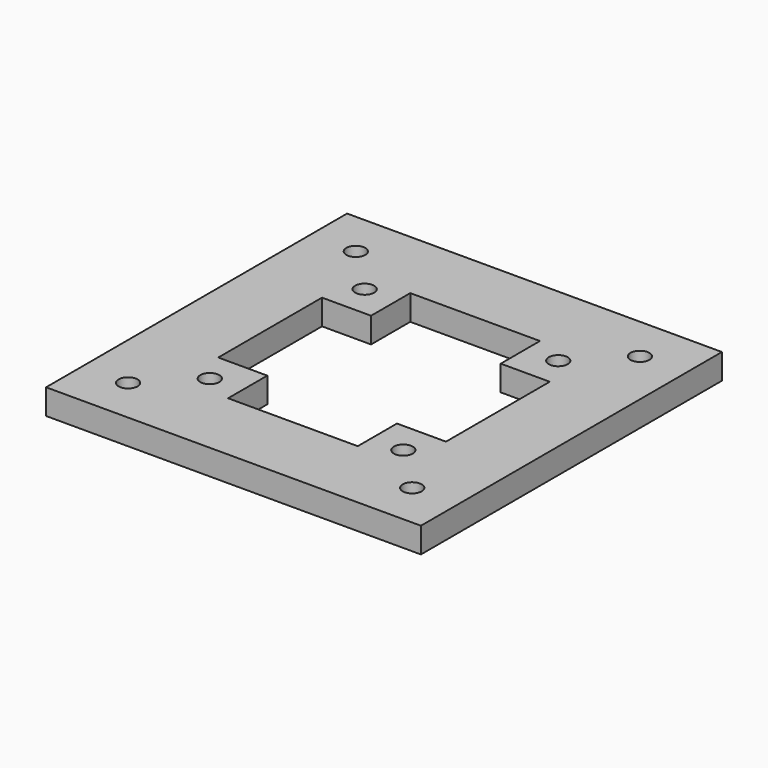
from build123d import *

# Parameters (mm, degrees)
F1_DEPTH = 2
F2_DEPTH = 4


with BuildPart() as f1:
    # F0 (on Top) → F1 (new body)
    with BuildSketch(Plane.XY):
        Polygon((0, -7.75), (0, -43.674267101), (7.675, -43.674267101), (7.675, -36), (7.675, -25.75), (7.675, -15.5), (7.675, -7.75), align=None)
        with BuildLine():
            Line((0, 0), (0, -7.75))
            Line((0, -7.75), (7.675, -7.75))
            Line((7.675, -7.75), (4.2740389016, -4.3158047541))
            ThreePointArc((4.2740389016, -4.3158047541), (2.152743633, -4.3054905145), (2.1630578726, -2.1841952459))
            Line((2.1630578726, -2.1841952459), (0, 0))
        make_face()
        with BuildLine():
            Line((7.675, 0), (0, 0))
            Line((0, 0), (2.1630578726, -2.1841952459))
            ThreePointArc((2.1630578726, -2.1841952459), (3.7959409001, -1.8655803072), (4.7185483871, -3.25))
            ThreePointArc((4.7185483871, -3.25), (4.6029680799, -3.827392513), (4.2740389016, -4.3158047541))
            Line((4.2740389016, -4.3158047541), (7.675, -7.75))
            Line((7.675, -7.75), (7.675, 0))
        make_face()
        Polygon((7.675, 0), (7.675, -7.75), (15.425, -7.75), (25.675, -7.75), (35.925, -7.75), (43.6, -7.75), (43.6, 0), align=None)
        Polygon((43.675, -36), (43.675, -43.75), (51.35, -43.75), (51.35, -7.825732899), (43.675, -7.825732899), (43.675, -15.5), (43.675, -25.75), align=None)
        Polygon((43.6, -7.825732899), (43.675, -7.825732899), (43.675, -7.75), (43.6, -7.825), align=None)
        with BuildLine():
            Line((51.35, -7.825732899), (51.35, 0))
            Line((51.35, 0), (49.1869421274, -2.1841952459))
            ThreePointArc((49.1869421274, -2.1841952459), (49.5158713057, -2.672607487), (49.6314516129, -3.25))
            ThreePointArc((49.6314516129, -3.25), (48.7088441259, -4.6344196928), (47.0759610984, -4.3158047541))
            Line((47.0759610984, -4.3158047541), (43.675, -7.75))
            Line((43.675, -7.75), (43.675, -7.825732899))
            Line((43.675, -7.825732899), (51.35, -7.825732899))
        make_face()
        with BuildLine():
            Line((49.1869421274, -2.1841952459), (51.35, 0))
            Line((51.35, 0), (43.6, 0))
            Line((43.6, 0), (43.6, -7.75))
            Line((43.6, -7.75), (43.675, -7.75))
            Line((43.675, -7.75), (47.0759610984, -4.3158047541))
            ThreePointArc((47.0759610984, -4.3158047541), (47.0656468588, -2.1945094855), (49.1869421274, -2.1841952459))
        make_face()
        with BuildLine():
            Line((9.3143398282, -9.3893398282), (7.675, -7.75))
            Line((7.675, -7.75), (7.675, -15.5))
            Line((7.675, -15.5), (11.55, -11.625))
            Line((11.55, -11.625), (11.4356601718, -11.5106601718))
            ThreePointArc((11.4356601718, -11.5106601718), (9.3143398282, -11.5106601718), (9.3143398282, -9.3893398282))
        make_face()
        Polygon((11.55, -11.625), (7.675, -15.5), (15.425, -15.5), align=None)
        Polygon((15.425, -15.5), (15.425, -7.75), (11.55, -11.625), align=None)
        with BuildLine():
            Line((15.425, -7.75), (7.675, -7.75))
            Line((7.675, -7.75), (9.3143398282, -9.3893398282))
            ThreePointArc((9.3143398282, -9.3893398282), (10.9490251485, -9.0641807012), (11.875, -10.45))
            ThreePointArc((11.875, -10.45), (11.7608192988, -11.0240251485), (11.4356601718, -11.5106601718))
            Line((11.4356601718, -11.5106601718), (11.55, -11.625))
            Line((11.55, -11.625), (15.425, -7.75))
        make_face()
        Polygon((39.8, -39.875), (43.675, -36), (35.925, -36), align=None)
        Polygon((35.925, -36), (35.925, -43.75), (39.8, -39.875), align=None)
        with BuildLine():
            Line((35.925, -43.75), (43.675, -43.75))
            Line((43.675, -43.75), (42.0356601718, -42.1106601718))
            ThreePointArc((42.0356601718, -42.1106601718), (39.9143398282, -42.1106601718), (39.9143398282, -39.9893398282))
            Line((39.9143398282, -39.9893398282), (39.8, -39.875))
            Line((39.8, -39.875), (35.925, -43.75))
        make_face()
        Polygon((7.75, -43.75), (7.75, -51.5), (43.675, -51.5), (43.675, -43.75), (35.925, -43.75), (25.675, -43.75), (15.425, -43.75), align=None)
        with BuildLine():
            Line((42.0356601718, -42.1106601718), (43.675, -43.75))
            Line((43.675, -43.75), (43.675, -36))
            Line((43.675, -36), (39.8, -39.875))
            Line((39.8, -39.875), (39.9143398282, -39.9893398282))
            ThreePointArc((39.9143398282, -39.9893398282), (41.5490251485, -39.6641807012), (42.475, -41.05))
            ThreePointArc((42.475, -41.05), (42.3608192988, -41.6240251485), (42.0356601718, -42.1106601718))
        make_face()
        Polygon((7.675, -43.75), (7.75, -43.75), (7.75, -43.675), align=None)
        with BuildLine():
            Line((7.75, -43.675), (7.75, -43.75))
            Line((7.75, -43.75), (15.425, -43.75))
            Line((15.425, -43.75), (11.55, -39.875))
            Line((11.55, -39.875), (11.4356601718, -39.9893398282))
            ThreePointArc((11.4356601718, -39.9893398282), (11.7608192988, -40.4759748515), (11.875, -41.05))
            ThreePointArc((11.875, -41.05), (10.9490251485, -42.4358192988), (9.3143398282, -42.1106601718))
            Line((9.3143398282, -42.1106601718), (7.75, -43.675))
        make_face()
        Polygon((7.75, -43.674267101), (7.675, -43.674267101), (7.675, -43.75), (7.75, -43.675), align=None)
        with BuildLine():
            Line((7.675, -36), (7.675, -43.674267101))
            Line((7.675, -43.674267101), (7.75, -43.674267101))
            Line((7.75, -43.674267101), (7.75, -43.675))
            Line((7.75, -43.675), (9.3143398282, -42.1106601718))
            ThreePointArc((9.3143398282, -42.1106601718), (9.3143398282, -39.9893398282), (11.4356601718, -39.9893398282))
            Line((11.4356601718, -39.9893398282), (11.55, -39.875))
            Line((11.55, -39.875), (7.675, -36))
        make_face()
        with BuildLine():
            Line((0, -43.674267101), (0, -51.5))
            Line((0, -51.5), (2.1630578726, -49.3158047541))
            ThreePointArc((2.1630578726, -49.3158047541), (2.152743633, -47.1945094855), (4.2740389016, -47.1841952459))
            Line((4.2740389016, -47.1841952459), (7.675, -43.75))
            Line((7.675, -43.75), (7.675, -43.674267101))
            Line((7.675, -43.674267101), (0, -43.674267101))
        make_face()
        with BuildLine():
            Line((2.1630578726, -49.3158047541), (0, -51.5))
            Line((0, -51.5), (7.75, -51.5))
            Line((7.75, -51.5), (7.75, -43.75))
            Line((7.75, -43.75), (7.675, -43.75))
            Line((7.675, -43.75), (4.2740389016, -47.1841952459))
            ThreePointArc((4.2740389016, -47.1841952459), (4.6029680799, -47.672607487), (4.7185483871, -48.25))
            ThreePointArc((4.7185483871, -48.25), (3.7959409001, -49.6344196928), (2.1630578726, -49.3158047541))
        make_face()
        with BuildLine():
            Line((43.675, -43.75), (43.675, -51.5))
            Line((43.675, -51.5), (51.35, -51.5))
            Line((51.35, -51.5), (49.1869421274, -49.3158047541))
            ThreePointArc((49.1869421274, -49.3158047541), (47.0656468588, -49.3054905145), (47.0759610984, -47.1841952459))
            Line((47.0759610984, -47.1841952459), (43.675, -43.75))
        make_face()
        with BuildLine():
            Line((49.1869421274, -49.3158047541), (51.35, -51.5))
            Line((51.35, -51.5), (51.35, -43.75))
            Line((51.35, -43.75), (43.675, -43.75))
            Line((43.675, -43.75), (47.0759610984, -47.1841952459))
            ThreePointArc((47.0759610984, -47.1841952459), (48.7088441259, -46.8655803072), (49.6314516129, -48.25))
            ThreePointArc((49.6314516129, -48.25), (49.5158713057, -48.827392513), (49.1869421274, -49.3158047541))
        make_face()
        Polygon((15.425, -36), (7.675, -36), (11.55, -39.875), align=None)
        Polygon((11.55, -39.875), (15.425, -43.75), (15.425, -36), align=None)
        Polygon((39.8, -11.625), (35.925, -7.75), (35.925, -15.5), align=None)
        Polygon((35.925, -15.5), (43.675, -15.5), (39.8, -11.625), align=None)
        with BuildLine():
            Line((43.6, -7.825), (43.6, -7.75))
            Line((43.6, -7.75), (35.925, -7.75))
            Line((35.925, -7.75), (39.8, -11.625))
            Line((39.8, -11.625), (39.9143398282, -11.5106601718))
            ThreePointArc((39.9143398282, -11.5106601718), (39.9143398282, -9.3893398282), (42.0356601718, -9.3893398282))
            Line((42.0356601718, -9.3893398282), (43.6, -7.825))
        make_face()
        with BuildLine():
            Line((43.675, -15.5), (43.675, -7.825732899))
            Line((43.675, -7.825732899), (43.6, -7.825732899))
            Line((43.6, -7.825732899), (43.6, -7.825))
            Line((43.6, -7.825), (42.0356601718, -9.3893398282))
            ThreePointArc((42.0356601718, -9.3893398282), (42.3608192988, -9.8759748515), (42.475, -10.45))
            ThreePointArc((42.475, -10.45), (41.5490251485, -11.8358192988), (39.9143398282, -11.5106601718))
            Line((39.9143398282, -11.5106601718), (39.8, -11.625))
            Line((39.8, -11.625), (43.675, -15.5))
        make_face()
    extrude(amount=F1_DEPTH)

    # F0 (on Top) → F2 (join)
    with BuildSketch(Plane.XY):
        with BuildLine():
            Line((2.1630578726, -49.3158047541), (0, -51.5))
            Line((0, -51.5), (7.75, -51.5))
            Line((7.75, -51.5), (7.75, -43.75))
            Line((7.75, -43.75), (7.675, -43.75))
            Line((7.675, -43.75), (4.2740389016, -47.1841952459))
            ThreePointArc((4.2740389016, -47.1841952459), (4.6029680799, -47.672607487), (4.7185483871, -48.25))
            ThreePointArc((4.7185483871, -48.25), (3.7959409001, -49.6344196928), (2.1630578726, -49.3158047541))
        make_face()
        Polygon((-3.95, -55.4885993485), (0, -51.5), (0, -43.674267101), (0, -7.75), (0, 0), (-3.95, 3.9885993485), align=None)
        with BuildLine():
            Line((0, -43.674267101), (0, -51.5))
            Line((0, -51.5), (2.1630578726, -49.3158047541))
            ThreePointArc((2.1630578726, -49.3158047541), (2.152743633, -47.1945094855), (4.2740389016, -47.1841952459))
            Line((4.2740389016, -47.1841952459), (7.675, -43.75))
            Line((7.675, -43.75), (7.675, -43.674267101))
            Line((7.675, -43.674267101), (0, -43.674267101))
        make_face()
        Polygon((7.75, -51.5), (0, -51.5), (-3.95, -55.4885993485), (55.3, -55.4885993485), (51.35, -51.5), (43.675, -51.5), align=None)
        Polygon((7.75, -43.75), (7.75, -51.5), (43.675, -51.5), (43.675, -43.75), (35.925, -43.75), (25.675, -43.75), (15.425, -43.75), align=None)
        Polygon((0, -7.75), (0, -43.674267101), (7.675, -43.674267101), (7.675, -36), (7.675, -25.75), (7.675, -15.5), (7.675, -7.75), align=None)
        with BuildLine():
            Line((43.675, -43.75), (43.675, -51.5))
            Line((43.675, -51.5), (51.35, -51.5))
            Line((51.35, -51.5), (49.1869421274, -49.3158047541))
            ThreePointArc((49.1869421274, -49.3158047541), (47.0656468588, -49.3054905145), (47.0759610984, -47.1841952459))
            Line((47.0759610984, -47.1841952459), (43.675, -43.75))
        make_face()
        with BuildLine():
            Line((7.75, -43.675), (7.75, -43.75))
            Line((7.75, -43.75), (15.425, -43.75))
            Line((15.425, -43.75), (11.55, -39.875))
            Line((11.55, -39.875), (11.4356601718, -39.9893398282))
            ThreePointArc((11.4356601718, -39.9893398282), (11.7608192988, -40.4759748515), (11.875, -41.05))
            ThreePointArc((11.875, -41.05), (10.9490251485, -42.4358192988), (9.3143398282, -42.1106601718))
            Line((9.3143398282, -42.1106601718), (7.75, -43.675))
        make_face()
        Polygon((7.675, -43.75), (7.75, -43.75), (7.75, -43.675), align=None)
        with BuildLine():
            Line((0, 0), (0, -7.75))
            Line((0, -7.75), (7.675, -7.75))
            Line((7.675, -7.75), (4.2740389016, -4.3158047541))
            ThreePointArc((4.2740389016, -4.3158047541), (2.152743633, -4.3054905145), (2.1630578726, -2.1841952459))
            Line((2.1630578726, -2.1841952459), (0, 0))
        make_face()
        Polygon((7.75, -43.674267101), (7.675, -43.674267101), (7.675, -43.75), (7.75, -43.675), align=None)
        with BuildLine():
            Line((7.675, -36), (7.675, -43.674267101))
            Line((7.675, -43.674267101), (7.75, -43.674267101))
            Line((7.75, -43.674267101), (7.75, -43.675))
            Line((7.75, -43.675), (9.3143398282, -42.1106601718))
            ThreePointArc((9.3143398282, -42.1106601718), (9.3143398282, -39.9893398282), (11.4356601718, -39.9893398282))
            Line((11.4356601718, -39.9893398282), (11.55, -39.875))
            Line((11.55, -39.875), (7.675, -36))
        make_face()
        Polygon((51.35, -51.5), (55.3, -55.4885993485), (55.3, 3.9885993485), (51.35, 0), (51.35, -7.825732899), (51.35, -43.75), align=None)
        Polygon((55.3, 3.9885993485), (-3.95, 3.9885993485), (0, 0), (7.675, 0), (43.6, 0), (51.35, 0), align=None)
        with BuildLine():
            Line((49.1869421274, -49.3158047541), (51.35, -51.5))
            Line((51.35, -51.5), (51.35, -43.75))
            Line((51.35, -43.75), (43.675, -43.75))
            Line((43.675, -43.75), (47.0759610984, -47.1841952459))
            ThreePointArc((47.0759610984, -47.1841952459), (48.7088441259, -46.8655803072), (49.6314516129, -48.25))
            ThreePointArc((49.6314516129, -48.25), (49.5158713057, -48.827392513), (49.1869421274, -49.3158047541))
        make_face()
        with BuildLine():
            Line((42.0356601718, -42.1106601718), (43.675, -43.75))
            Line((43.675, -43.75), (43.675, -36))
            Line((43.675, -36), (39.8, -39.875))
            Line((39.8, -39.875), (39.9143398282, -39.9893398282))
            ThreePointArc((39.9143398282, -39.9893398282), (41.5490251485, -39.6641807012), (42.475, -41.05))
            ThreePointArc((42.475, -41.05), (42.3608192988, -41.6240251485), (42.0356601718, -42.1106601718))
        make_face()
        with BuildLine():
            Line((35.925, -43.75), (43.675, -43.75))
            Line((43.675, -43.75), (42.0356601718, -42.1106601718))
            ThreePointArc((42.0356601718, -42.1106601718), (39.9143398282, -42.1106601718), (39.9143398282, -39.9893398282))
            Line((39.9143398282, -39.9893398282), (39.8, -39.875))
            Line((39.8, -39.875), (35.925, -43.75))
        make_face()
        Polygon((43.675, -36), (43.675, -43.75), (51.35, -43.75), (51.35, -7.825732899), (43.675, -7.825732899), (43.675, -15.5), (43.675, -25.75), align=None)
        Polygon((11.55, -39.875), (15.425, -43.75), (15.425, -36), align=None)
        with BuildLine():
            Line((7.675, 0), (0, 0))
            Line((0, 0), (2.1630578726, -2.1841952459))
            ThreePointArc((2.1630578726, -2.1841952459), (3.7959409001, -1.8655803072), (4.7185483871, -3.25))
            ThreePointArc((4.7185483871, -3.25), (4.6029680799, -3.827392513), (4.2740389016, -4.3158047541))
            Line((4.2740389016, -4.3158047541), (7.675, -7.75))
            Line((7.675, -7.75), (7.675, 0))
        make_face()
        Polygon((7.675, 0), (7.675, -7.75), (15.425, -7.75), (25.675, -7.75), (35.925, -7.75), (43.6, -7.75), (43.6, 0), align=None)
        with BuildLine():
            Line((9.3143398282, -9.3893398282), (7.675, -7.75))
            Line((7.675, -7.75), (7.675, -15.5))
            Line((7.675, -15.5), (11.55, -11.625))
            Line((11.55, -11.625), (11.4356601718, -11.5106601718))
            ThreePointArc((11.4356601718, -11.5106601718), (9.3143398282, -11.5106601718), (9.3143398282, -9.3893398282))
        make_face()
        with BuildLine():
            Line((15.425, -7.75), (7.675, -7.75))
            Line((7.675, -7.75), (9.3143398282, -9.3893398282))
            ThreePointArc((9.3143398282, -9.3893398282), (10.9490251485, -9.0641807012), (11.875, -10.45))
            ThreePointArc((11.875, -10.45), (11.7608192988, -11.0240251485), (11.4356601718, -11.5106601718))
            Line((11.4356601718, -11.5106601718), (11.55, -11.625))
            Line((11.55, -11.625), (15.425, -7.75))
        make_face()
        Polygon((15.425, -36), (7.675, -36), (11.55, -39.875), align=None)
        Polygon((35.925, -36), (35.925, -43.75), (39.8, -39.875), align=None)
        Polygon((39.8, -39.875), (43.675, -36), (35.925, -36), align=None)
        Polygon((15.425, -15.5), (15.425, -7.75), (11.55, -11.625), align=None)
        Polygon((11.55, -11.625), (7.675, -15.5), (15.425, -15.5), align=None)
        with BuildLine():
            Line((49.1869421274, -2.1841952459), (51.35, 0))
            Line((51.35, 0), (43.6, 0))
            Line((43.6, 0), (43.6, -7.75))
            Line((43.6, -7.75), (43.675, -7.75))
            Line((43.675, -7.75), (47.0759610984, -4.3158047541))
            ThreePointArc((47.0759610984, -4.3158047541), (47.0656468588, -2.1945094855), (49.1869421274, -2.1841952459))
        make_face()
        with BuildLine():
            Line((51.35, -7.825732899), (51.35, 0))
            Line((51.35, 0), (49.1869421274, -2.1841952459))
            ThreePointArc((49.1869421274, -2.1841952459), (49.5158713057, -2.672607487), (49.6314516129, -3.25))
            ThreePointArc((49.6314516129, -3.25), (48.7088441259, -4.6344196928), (47.0759610984, -4.3158047541))
            Line((47.0759610984, -4.3158047541), (43.675, -7.75))
            Line((43.675, -7.75), (43.675, -7.825732899))
            Line((43.675, -7.825732899), (51.35, -7.825732899))
        make_face()
        Polygon((43.6, -7.825732899), (43.675, -7.825732899), (43.675, -7.75), (43.6, -7.825), align=None)
        with BuildLine():
            Line((43.675, -15.5), (43.675, -7.825732899))
            Line((43.675, -7.825732899), (43.6, -7.825732899))
            Line((43.6, -7.825732899), (43.6, -7.825))
            Line((43.6, -7.825), (42.0356601718, -9.3893398282))
            ThreePointArc((42.0356601718, -9.3893398282), (42.3608192988, -9.8759748515), (42.475, -10.45))
            ThreePointArc((42.475, -10.45), (41.5490251485, -11.8358192988), (39.9143398282, -11.5106601718))
            Line((39.9143398282, -11.5106601718), (39.8, -11.625))
            Line((39.8, -11.625), (43.675, -15.5))
        make_face()
        Polygon((35.925, -15.5), (43.675, -15.5), (39.8, -11.625), align=None)
        with BuildLine():
            Line((43.6, -7.825), (43.6, -7.75))
            Line((43.6, -7.75), (35.925, -7.75))
            Line((35.925, -7.75), (39.8, -11.625))
            Line((39.8, -11.625), (39.9143398282, -11.5106601718))
            ThreePointArc((39.9143398282, -11.5106601718), (39.9143398282, -9.3893398282), (42.0356601718, -9.3893398282))
            Line((42.0356601718, -9.3893398282), (43.6, -7.825))
        make_face()
        Polygon((43.675, -7.75), (43.6, -7.75), (43.6, -7.825), align=None)
        Polygon((39.8, -11.625), (35.925, -7.75), (35.925, -15.5), align=None)
    extrude(amount=F2_DEPTH)


solid = f1.part
